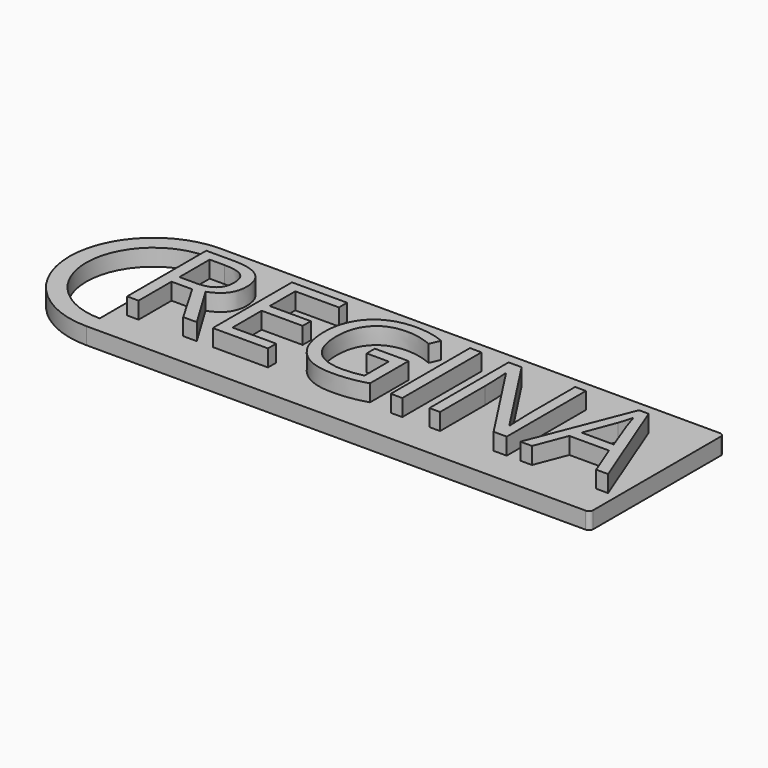
from build123d import *

# Parameters (mm, degrees)
F4_DEPTH     = 2
F1_TEXT_SIZE = 16.5175498968
F2_DEPTH     = 2
F3_R         = 0.5


# Not quite as in the source:
# - Text() gives the source's letters only with a copy of the font that has no kerning and outlines rounded to 1/6400 em; it was checked with that copy


with BuildPart() as f4:
    # F0 (on Top) → F4 (new body)
    with BuildSketch(Plane.XY):
        Polygon((54.7291392038, 3.2207785361), (-5.2708607962, 3.2207785361), (-5.2708607962, 1.2207785361), (-5.2708607962, -14.7792214639), (-5.2708607962, -16.7792214639), (54.7291392038, -16.7792214639), align=None)
        with BuildLine():
            Line((-5.2708607962, 1.2207785361), (-5.2708607962, 3.2207785361))
            ThreePointArc((-5.2708607962, 3.2207785361), (-15.2708607962, -6.7792214639), (-5.2708607962, -16.7792214639))
            Line((-5.2708607962, -16.7792214639), (-5.2708607962, -14.7792214639))
            ThreePointArc((-5.2708607962, -14.7792214639), (-13.2708607962, -6.7792214639), (-5.2708607962, 1.2207785361))
        make_face()
    extrude(amount=F4_DEPTH)

    # F1 (on face) → F2 (join)
    with BuildSketch(Plane.XY.offset(2)):
        with Locations((-5.2708607962, -12.7255394268)):
            Text('REGINA', F1_TEXT_SIZE, font='Open Sans', text_align=(TextAlign.LEFT, TextAlign.BOTTOM))
    extrude(amount=F2_DEPTH)

    # F3
    f3_edges = [f4.edges().sort_by_distance(p)[0] for p in [
        (54.729139, -16.779221, 1),
        (54.729139, 3.220779, 1),
    ]]
    fillet(f3_edges, radius=F3_R)


solid = f4.part
